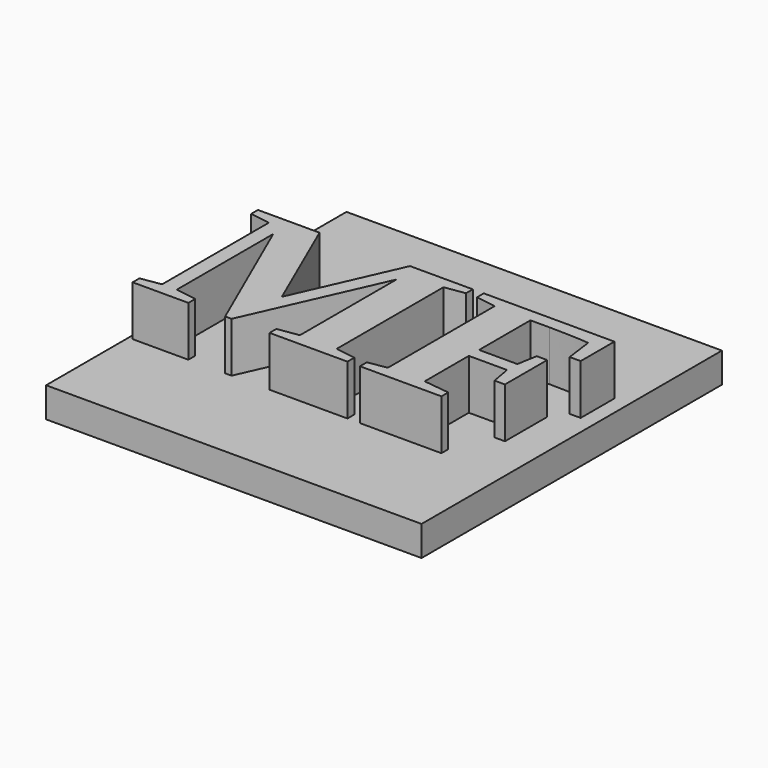
from build123d import *

# Parameters (mm, degrees)
F0_W         = 15
F0_H         = 15
F1_DEPTH     = 1.2
F2_TEXT_SIZE = 9.5579450418
F3_DEPTH     = 2


# Not quite as in the source:
# - Text() gives the source's letters only with a copy of the font that has no kerning and outlines rounded to 1/6400 em; it was checked with that copy


with BuildPart() as f1:
    # F0 (on Top) → F1 (new body)
    with BuildSketch(Plane.XY):
        with Locations((7.5, 7.5)):
            Rectangle(F0_W, F0_H)
    extrude(amount=F1_DEPTH)

    # F2 (on face) → F3 (join)
    with BuildSketch(Plane.XY.offset(1.2)):
        with Locations((0, 4.1182795699)):
            Text('MF', F2_TEXT_SIZE, font='Tinos', font_style=FontStyle.BOLD, text_align=(TextAlign.LEFT, TextAlign.BOTTOM))
    extrude(amount=F3_DEPTH)


solid = f1.part
